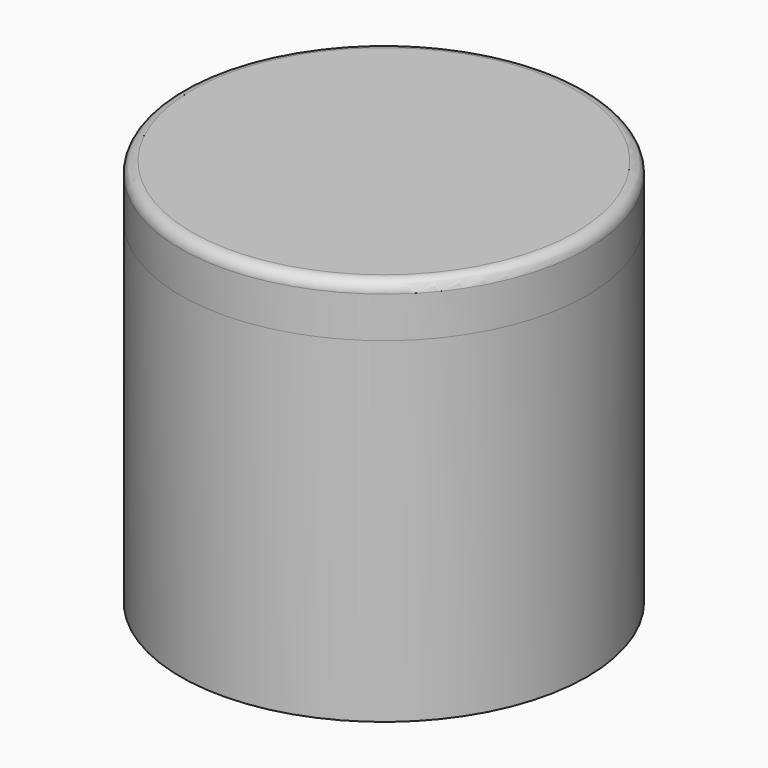
from build123d import *

# Parameters (mm, degrees)
F0_R     = 54.5
F1_DEPTH = 90
F0_W     = 7
F0_H     = 7
F2_DEPTH = 4
F3_R     = 54.5
F3_R_2   = 51.5
F4_DEPTH = 11
F5_R     = 54.5
F5_R_2   = 51.5
F5_R_3   = 48.5912547039
F6_DEPTH = 3
F7_R     = 3


# Not quite as in the source:
# - a feature of the source that left no trace in its solid (it failed there, or was rolled back) is left out


with BuildPart() as f1:
    # F0 (on Top) → F1 (new body)
    with BuildSketch(Plane.XY):
        Circle(F0_R)
        with BuildLine():
            ThreePointArc((50.3785668712, 3.5), (50.4696325873, 1.7510529693), (50.5, 0))
            ThreePointArc((50.5, 0), (50.4696325873, -1.7510529693), (50.3785668712, -3.5))
            ThreePointArc((50.3785668712, -3.5), (35.7088924499, -35.7088924499), (3.5, -50.3785668712))
            ThreePointArc((3.5, -50.3785668712), (0, -50.5), (-3.5, -50.3785668712))
            ThreePointArc((-3.5, -50.3785668712), (-35.7088924499, -35.7088924499), (-50.3785668712, -3.5))
            ThreePointArc((-50.3785668712, -3.5), (-50.5, 0), (-50.3785668712, 3.5))
            ThreePointArc((-50.3785668712, 3.5), (-35.7088924499, 35.7088924499), (-3.5, 50.3785668712))
            ThreePointArc((-3.5, 50.3785668712), (0, 50.5), (3.5, 50.3785668712))
            ThreePointArc((3.5, 50.3785668712), (35.7088924499, 35.7088924499), (50.3785668712, 3.5))
        make_face(mode=Mode.SUBTRACT)
    extrude(amount=F1_DEPTH)

    # F0 (on Top) → F2 (join)
    with BuildSketch(Plane.XY):
        Rectangle(F0_W, F0_H)
        with BuildLine():
            ThreePointArc((-3.5, -50.3785668712), (0, -50.5), (3.5, -50.3785668712))
            Line((3.5, -50.3785668712), (3.5, -3.5))
            Line((3.5, -3.5), (-3.5, -3.5))
            Line((-3.5, -3.5), (-3.5, -50.3785668712))
        make_face()
        with BuildLine():
            ThreePointArc((50.3785668712, -3.5), (50.4696325873, -1.7510529693), (50.5, 0))
            ThreePointArc((50.5, 0), (50.4696325873, 1.7510529693), (50.3785668712, 3.5))
            Line((50.3785668712, 3.5), (3.5, 3.5))
            Line((3.5, 3.5), (3.5, -3.5))
            Line((3.5, -3.5), (50.3785668712, -3.5))
        make_face()
        with BuildLine():
            Line((3.5, 3.5), (3.5, 50.3785668712))
            ThreePointArc((3.5, 50.3785668712), (0, 50.5), (-3.5, 50.3785668712))
            Line((-3.5, 50.3785668712), (-3.5, 3.5))
            Line((-3.5, 3.5), (3.5, 3.5))
        make_face()
        with BuildLine():
            Line((-3.5, -3.5), (-3.5, 3.5))
            Line((-3.5, 3.5), (-50.3785668712, 3.5))
            ThreePointArc((-50.3785668712, 3.5), (-50.5, 0), (-50.3785668712, -3.5))
            Line((-50.3785668712, -3.5), (-3.5, -3.5))
        make_face()
    extrude(amount=F2_DEPTH)


with BuildPart() as f4:
    # F3 (on face) → F4 (new body)
    with BuildSketch(Plane.XY.offset(90)):
        Circle(F3_R)
        Circle(F3_R_2, mode=Mode.SUBTRACT)
    extrude(amount=F4_DEPTH)

    # F5 (on face) → F6 (join)
    with BuildSketch(Plane.XY.offset(101)):
        Circle(F5_R)
        Circle(F5_R_2, mode=Mode.SUBTRACT)
        Circle(F5_R_2)
        Circle(F5_R_3, mode=Mode.SUBTRACT)
        Circle(F5_R_3)
    extrude(amount=F6_DEPTH)

    # F7
    f7_edges = [f4.edges().sort_by_distance(p)[0] for p in [
        (-54.5, 0, 104),
    ]]
    fillet(f7_edges, radius=F7_R)


solid = Compound([f1.part, f4.part])
